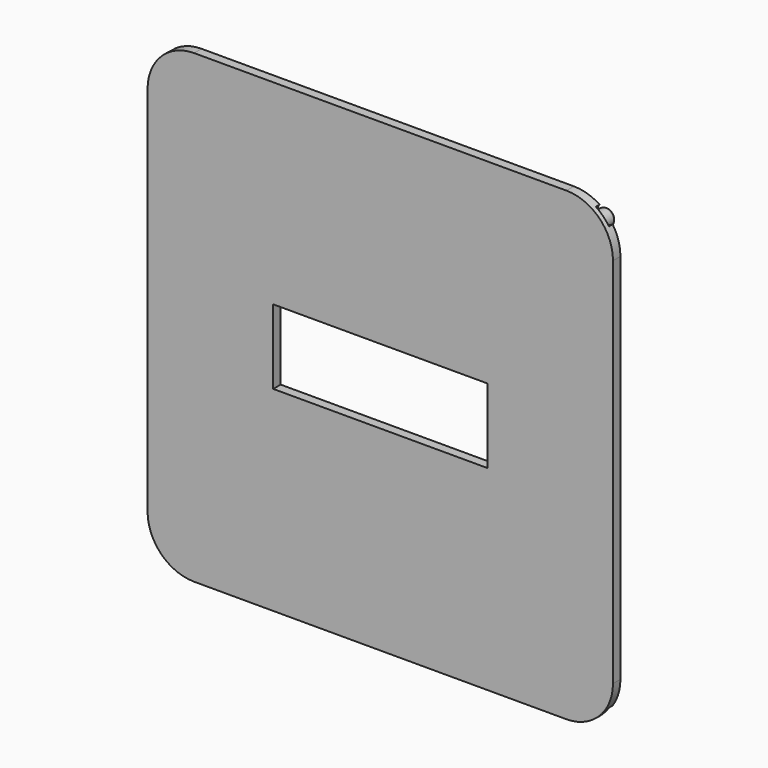
from build123d import *

# Parameters (mm, degrees)
F0_W     = 46
F0_H     = 16
F1_DEPTH = 2
F2_R     = 1.9
F3_DEPTH = 4
F3_TAPER = 2
F5_DEPTH = 1
F6_R     = 0.6


# Not quite as in the source:
# - a feature names something its author has since deleted; it is built from what else it names


with BuildPart() as f1:
    # F0 (on Front) → F1 (new body)
    with BuildSketch(Plane.XZ):
        Polygon((-40, -50), (40, -50), (40, -40), (50, -40), (50, 40), (40, 40), (40, 50), (-40, 50), (-40, 40), (-50, 40), (-50, -40), (-40, -40), align=None)
        Rectangle(F0_W, F0_H, mode=Mode.SUBTRACT)
        with BuildLine():
            Line((40, -40), (40, -50))
            ThreePointArc((40, -50), (47.0710678119, -47.0710678119), (50, -40))
            Line((50, -40), (40, -40))
        make_face()
        with BuildLine():
            ThreePointArc((-50, -40), (-47.0710678119, -47.0710678119), (-40, -50))
            Line((-40, -50), (-40, -40))
            Line((-40, -40), (-50, -40))
        make_face()
        with BuildLine():
            Line((40, 40), (50, 40))
            ThreePointArc((50, 40), (47.0710678119, 47.0710678119), (40, 50))
            Line((40, 50), (40, 40))
        make_face()
        with BuildLine():
            ThreePointArc((-40, 50), (-47.0710678119, 47.0710678119), (-50, 40))
            Line((-50, 40), (-40, 40))
            Line((-40, 40), (-40, 50))
        make_face()
    extrude(amount=F1_DEPTH)

    # F2 (on face) → F3 (join)
    with BuildSketch(Plane(origin=(0, 0, 0), x_dir=(-1, 0, 0), z_dir=(0, 1, 0))):
        with Locations((-44, 44)):
            Circle(F2_R)
        with Locations((44, 44)):
            Circle(F2_R)
        with Locations((-44, -44)):
            Circle(F2_R)
        with Locations((44, -44)):
            Circle(F2_R)
    extrude(amount=F3_DEPTH, taper=F3_TAPER)

    # F4 (on face) → F5 (cut)
    with BuildSketch(Plane.XZ):
        with BuildLine():
            ThreePointArc((48.3367711836, 45.5225217277), (47.0710678119, 47.0710678119), (45.5225217277, 48.3367711836))
            ThreePointArc((45.5225217277, 48.3367711836), (45.6568542495, 45.6568542495), (48.3367711836, 45.5225217277))
        make_face()
        with BuildLine():
            ThreePointArc((-48.3367711836, 45.5225217277), (-45.6568542495, 45.6568542495), (-45.5225217277, 48.3367711836))
            ThreePointArc((-45.5225217277, 48.3367711836), (-47.0710678119, 47.0710678119), (-48.3367711836, 45.5225217277))
        make_face()
        with BuildLine():
            ThreePointArc((-48.3367711836, -45.5225217277), (-47.0710678119, -47.0710678119), (-45.5225217277, -48.3367711836))
            ThreePointArc((-45.5225217277, -48.3367711836), (-45.6568542495, -45.6568542495), (-48.3367711836, -45.5225217277))
        make_face()
        with BuildLine():
            ThreePointArc((48.3367711836, -45.5225217277), (45.6568542495, -45.6568542495), (45.5225217277, -48.3367711836))
            ThreePointArc((45.5225217277, -48.3367711836), (47.0710678119, -47.0710678119), (48.3367711836, -45.5225217277))
        make_face()
    extrude(amount=F5_DEPTH, mode=Mode.SUBTRACT)

    # F6
    f6_edges = [f1.edges().sort_by_distance(p)[0] for p in [
        (45.760317, 4, 44),
        (45.760317, 4, -44),
        (-42.239683, 4, 44),
        (-42.239683, 4, -44),
    ]]
    fillet(f6_edges, radius=F6_R)


solid = f1.part
